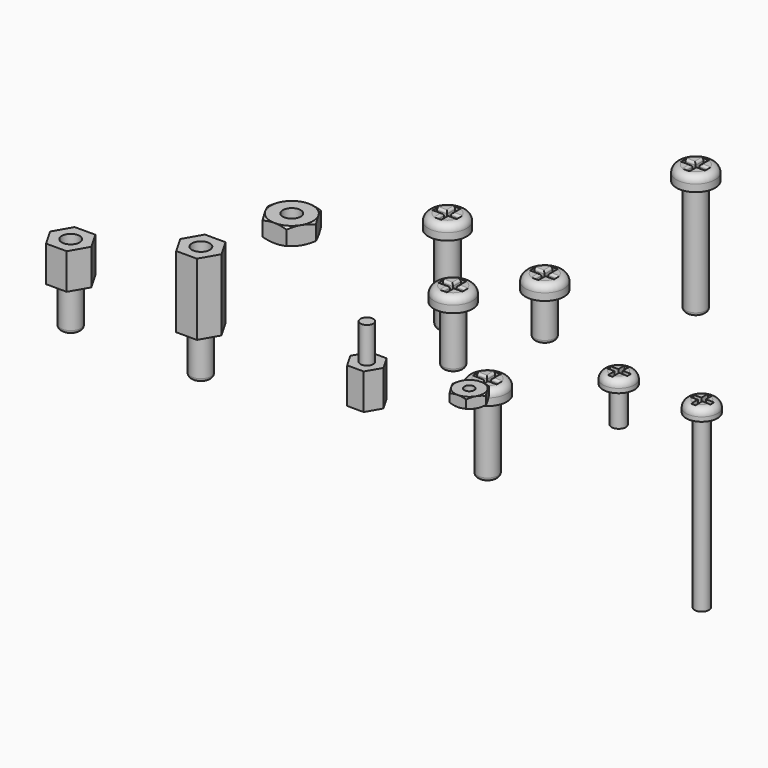
from build123d import *

# Parameters (mm, degrees)
F0_R        = 1.25
F1_DEPTH    = 2.5
F2_R        = 2.7
F3_DEPTH    = 2
F4_R        = 1
F6_DEPTH    = 1
F7_T1_DEPTH = 2.1580906364
F7_T3_DEPTH = 2.1580906364
F7_T5_DEPTH = 2.1580906364
F7_T7_DEPTH = 2.1580906364
F8_R        = 1.45
F13_DEPTH   = 12
F14_R       = 0.5
F15_R       = 1.45
F16_DEPTH   = 6
F17_R       = 0.5
F20_R       = 1.45
F21_DEPTH   = 10
F22_R       = 0.5
F23_R       = 1.45
F24_DEPTH   = 8
F25_R       = 0.5
F27_DEPTH   = 10
F28_R       = 1.25
F29_DEPTH   = 7.38
F30_R       = 1.45
F31_DEPTH   = 6
F32_R       = 0.5
F39_R       = 0.75
F40_DEPTH   = 5
F41_R       = 0.9
F41_R_2     = 0.75
F42_DEPTH   = 5
F43_R       = 0.7
F44_DEPTH   = 1.5
F45_R       = 2.2
F46_DEPTH   = 1.6
F48_DEPTH   = 1
F51_R       = 1
F52_DEPTH   = 5
F54_R       = 7.4954370555
F54_R_2     = 1.25
F55_DEPTH   = 5
F56_R       = 1
F57_DEPTH   = 24
F64_R       = 1.45
F65_DEPTH   = 16
F66_R       = 0.5


# Not quite as in the source:
# - a fillet or chamfer that OpenCascade refuses, or shapes differently, is made with other operations: its cross-section is extruded or revolved along the edge and cut away or added


with BuildPart() as f1:
    # F0 (on Top) → F1 (new body)
    with BuildSketch(Plane.XY):
        Polygon((-50.9010210277, 27.3592374967), (-49.1410704475, 30.2757263598), (-50.7868486027, 33.2581327032), (-54.1925773381, 33.3240501835), (-55.9525279183, 30.4075613204), (-54.3067497631, 27.425154977), align=None)
        with Locations((-52.5467991829, 30.3416438401)):
            Circle(F0_R, mode=Mode.SUBTRACT)
    extrude(amount=F1_DEPTH)

    # F37 (on 3pt) → F38 (revolve, cut)
    with BuildSketch(Plane(origin=(-0.6049917377, -1.0025575065, 0), x_dir=(-0.8561876086, 0.5166650549, 0), z_dir=(0.5166650549, 0.8561876086, 0))):
        Polygon((65.9979552705, 2.5), (63.6163854101, 2.5), (65.9979552705, 1.125), align=None)
        Polygon((65.9979552705, 0), (65.9979552705, 1.125), (63.6163854101, 0), align=None)
    revolve(axis=Axis((-52.5467991829, 30.3416438401, 2.5), (0, 0, 1)), mode=Mode.SUBTRACT)


with BuildPart() as f3:
    # F2 (on Top) → F3 (new body)
    with BuildSketch(Plane.XY):
        with Locations((-39.9160310626, 41.7706146836)):
            Circle(F2_R)
    extrude(amount=F3_DEPTH)

    # F4
    f4_edges = [f3.edges().sort_by_distance(p)[0] for p in [
        (-42.616031, 41.770615, 2),
    ]]
    fillet(f4_edges, radius=F4_R)

    # F5 (on face) → F6 (cut)
    with BuildSketch(Plane.XY.offset(2)):
        Polygon((-39.645745744, 43.4489906387), (-40.1863163812, 43.4489906387), (-40.1863163812, 42.0409000023), (-41.5944070177, 42.0409000023), (-41.5944070177, 41.500329365), (-40.1863163812, 41.500329365), (-40.1863163812, 40.0922387286), (-39.645745744, 40.0922387286), (-39.645745744, 41.500329365), (-38.2376551075, 41.500329365), (-38.2376551075, 42.0409000023), (-39.645745744, 42.0409000023), align=None)
    extrude(amount=-F6_DEPTH, mode=Mode.SUBTRACT)

    # F7: fillet of radius 0.3 on 8 edges, made by hand

    # F7_s2 → F7_t1 (cut)
    with BuildSketch(Plane.YZ.offset(-40.395745744)):
        with BuildLine():
            ThreePointArc((42.3409000023, 2), (42.1287679679, 1.9121320344), (42.0409000023, 1.7))
            Line((42.0409000023, 1.7), (42.0409000023, 2))
            Line((42.0409000023, 2), (42.3409000023, 2))
        make_face()
        with BuildLine():
            ThreePointArc((41.200329365, 2), (41.4124613994, 1.9121320344), (41.500329365, 1.7))
            Line((41.500329365, 1.7), (41.500329365, 2))
            Line((41.500329365, 2), (41.200329365, 2))
        make_face()
    extrude(amount=F7_T1_DEPTH, mode=Mode.SUBTRACT)

    # F7_s4 → F7_t3 (cut)
    with BuildSketch(Plane.XZ.offset(-43.4489906387)):
        with BuildLine():
            ThreePointArc((-39.345745744, 2), (-39.5578777783, 1.9121320344), (-39.645745744, 1.7))
            Line((-39.645745744, 1.7), (-39.645745744, 2))
            Line((-39.645745744, 2), (-39.345745744, 2))
        make_face()
        with BuildLine():
            ThreePointArc((-40.4863163812, 2), (-40.2741843469, 1.9121320344), (-40.1863163812, 1.7))
            Line((-40.1863163812, 1.7), (-40.1863163812, 2))
            Line((-40.1863163812, 2), (-40.4863163812, 2))
        make_face()
    extrude(amount=F7_T3_DEPTH, mode=Mode.SUBTRACT)

    # F7_s6 → F7_t5 (cut)
    with BuildSketch(Plane.YZ.offset(-41.5944070177)):
        with BuildLine():
            ThreePointArc((42.3409000023, 2), (42.1287679679, 1.9121320344), (42.0409000023, 1.7))
            Line((42.0409000023, 1.7), (42.0409000023, 2))
            Line((42.0409000023, 2), (42.3409000023, 2))
        make_face()
        with BuildLine():
            ThreePointArc((41.200329365, 2), (41.4124613994, 1.9121320344), (41.500329365, 1.7))
            Line((41.500329365, 1.7), (41.500329365, 2))
            Line((41.500329365, 2), (41.200329365, 2))
        make_face()
    extrude(amount=F7_T5_DEPTH, mode=Mode.SUBTRACT)

    # F7_s8 → F7_t7 (cut)
    with BuildSketch(Plane.XZ.offset(-42.250329365)):
        with BuildLine():
            ThreePointArc((-40.4863163812, 2), (-40.2741843469, 1.9121320344), (-40.1863163812, 1.7))
            Line((-40.1863163812, 1.7), (-40.1863163812, 2))
            Line((-40.1863163812, 2), (-40.4863163812, 2))
        make_face()
        with BuildLine():
            ThreePointArc((-39.345745744, 2), (-39.5578777783, 1.9121320344), (-39.645745744, 1.7))
            Line((-39.645745744, 1.7), (-39.645745744, 2))
            Line((-39.645745744, 2), (-39.345745744, 2))
        make_face()
    extrude(amount=F7_T7_DEPTH, mode=Mode.SUBTRACT)


with BuildPart() as f9_1:
    # F9: copy of F3
    add(f3.part.moved(Location((13.6, 0, -3))))


with BuildPart() as f10_1:
    # F10: copy of F9_1
    add(f9_1.part.moved(Location((-3.2, 30.4, 0))))

    # F64 (on face) → F65 (join)
    with BuildSketch(Plane(origin=(0, 0, -3), x_dir=(1, 0, 0), z_dir=(0, 0, -1))):
        with Locations((-29.5160310626, -72.1706146836)):
            Circle(F64_R)
    extrude(amount=F65_DEPTH)

    # F66
    f66_edges = [f10_1.edges().sort_by_distance(p)[0] for p in [
        (-30.966031, 72.170615, -19),
    ]]
    fillet(f66_edges, radius=F66_R)


with BuildPart() as f11_1:
    # F11: copy of F3
    add(f3.part.moved(Location((16.3, -46.7, 0))))


with BuildPart() as f12_1:
    # F12: copy of F3
    add(f3.part.moved(Location((11.2, -13, 0))))

    # F23 (on face) → F24 (join)
    with BuildSketch(Plane(origin=(0, 0, 0), x_dir=(1, 0, 0), z_dir=(0, 0, -1))):
        with Locations((-28.7160310626, -28.7706146836)):
            Circle(F23_R)
    extrude(amount=F24_DEPTH)

    # F25
    f25_edges = [f12_1.edges().sort_by_distance(p)[0] for p in [
        (-30.166031, 28.770615, -8),
    ]]
    fillet(f25_edges, radius=F25_R)


with BuildPart() as f3_1:
    add(f3.part)

    # F8 (on face) → F13 (join)
    with BuildSketch(Plane(origin=(0, 0, 0), x_dir=(1, 0, 0), z_dir=(0, 0, -1))):
        with Locations((-39.9160310626, -41.7706146836)):
            Circle(F8_R)
    extrude(amount=F13_DEPTH)

    # F14
    f14_edges = [f3_1.edges().sort_by_distance(p)[0] for p in [
        (-41.366031, 41.770615, -12),
    ]]
    fillet(f14_edges, radius=F14_R)


with BuildPart() as f9_1_1:
    add(f9_1.part)

    # F15 (on face) → F16 (join)
    with BuildSketch(Plane(origin=(0, 0, -3), x_dir=(1, 0, 0), z_dir=(0, 0, -1))):
        with Locations((-26.3160310626, -41.7706146836)):
            Circle(F15_R)
    extrude(amount=F16_DEPTH)

    # F17
    f17_edges = [f9_1_1.edges().sort_by_distance(p)[0] for p in [
        (-27.766031, 41.770615, -9),
    ]]
    fillet(f17_edges, radius=F17_R)


with BuildPart() as f11_1_1:
    # F18: moved
    add(f11_1.part.moved(Location((7.2, 0, 30.6))))


with BuildPart() as f11_1_2:
    # F19: moved
    add(f11_1_1.part.moved(Location((-1.9, 26.7, -35.8))))

    # F20 (on face) → F21 (join)
    with BuildSketch(Plane(origin=(0, 0, -5.2), x_dir=(1, 0, 0), z_dir=(0, 0, -1))):
        with Locations((-18.3160310626, -21.7706146836)):
            Circle(F20_R)
    extrude(amount=F21_DEPTH)

    # F22
    f22_edges = [f11_1_2.edges().sort_by_distance(p)[0] for p in [
        (-19.766031, 21.770615, -15.2),
    ]]
    fillet(f22_edges, radius=F22_R)


with BuildPart() as f27:
    # F26 (on Top) → F27 (new body)
    with BuildSketch(Plane.XY):
        Polygon((-44.9484995911, 4.2532703688), (-43.5051239182, 6.7532703688), (-44.9484995911, 9.2532703688), (-47.8352509371, 9.2532703688), (-49.2786266101, 6.7532703688), (-47.8352509371, 4.2532703688), align=None)
    extrude(amount=F27_DEPTH)

    # F28 (on face) → F29 (cut)
    with BuildSketch(Plane.XY.offset(10)):
        with Locations((-46.3918752641, 6.7532703688)):
            Circle(F28_R)
    extrude(amount=-F29_DEPTH, mode=Mode.SUBTRACT)

    # F30 (on face) → F31 (join)
    with BuildSketch(Plane(origin=(0, 0, 0), x_dir=(1, 0, 0), z_dir=(0, 0, -1))):
        with Locations((-46.3918752641, -6.7532703688)):
            Circle(F30_R)
    extrude(amount=F31_DEPTH)

    # F32
    f32_edges = [f27.edges().sort_by_distance(p)[0] for p in [
        (-47.841875, 6.75327, -6),
    ]]
    fillet(f32_edges, radius=F32_R)


with BuildPart() as f40:
    # F39 (on Top) → F40 (new body)
    with BuildSketch(Plane.XY):
        Polygon((-20.0601718143, 2.3061985367), (-18.9054712759, 4.3061985367), (-20.0601718143, 6.3061985367), (-22.3695728911, 6.3061985367), (-23.5242734295, 4.3061985367), (-22.3695728911, 2.3061985367), align=None)
        with Locations((-21.2148723527, 4.3061985367)):
            Circle(F39_R, mode=Mode.SUBTRACT)
    extrude(amount=F40_DEPTH)

    # F41 (on face) → F42 (join)
    with BuildSketch(Plane.XY.offset(5)):
        with Locations((-21.2148723527, 4.3061985367)):
            Circle(F41_R)
        with Locations((-21.2148723527, 4.3061985367)):
            Circle(F41_R_2, mode=Mode.SUBTRACT)
        with Locations((-21.2148723527, 4.3061985367)):
            Circle(F41_R_2)
    extrude(amount=F42_DEPTH)


with BuildPart() as f44:
    # F43 (on Top) → F44 (new body)
    with BuildSketch(Plane.XY):
        Polygon((-11.6123360878, 9.6400680006), (-10.4576355494, 11.6400680006), (-11.6123360878, 13.6400680006), (-13.9217371645, 13.6400680006), (-15.0764377029, 11.6400680006), (-13.9217371645, 9.6400680006), align=None)
        with Locations((-12.7670366262, 11.6400680006)):
            Circle(F43_R, mode=Mode.SUBTRACT)
    extrude(amount=F44_DEPTH)

    # F62 (on 3pt) → F63 (revolve, cut)
    with BuildSketch(Plane(origin=(-8.2320564517, 14.2583400251, 0), x_dir=(-0.8660254038, -0.5, 0), z_dir=(-0.5, 0.8660254038, 0))):
        Polygon((1.9375059433, 0.75), (3.236544049, 1.5), (1.9375059433, 1.5), align=None)
        Polygon((3.236544049, 0), (1.9375059433, 0.75), (1.9375059433, 0), align=None)
    revolve(axis=Axis((-12.7670366262, 11.6400680006, 1.5), (0, 0, 1)), mode=Mode.SUBTRACT)


with BuildPart() as f46:
    # F45 (on Top) → F46 (new body)
    with BuildSketch(Plane.XY):
        with Locations((-2.4725666735, 24.8899627477)):
            Circle(F45_R)
    extrude(amount=F46_DEPTH)

    # F47 (on face) → F48 (cut)
    with BuildSketch(Plane.XY.offset(1.6)):
        Polygon((-2.1590052638, 24.576401338), (-1.0345844785, 24.576401338), (-1.0345844785, 25.2035241574), (-2.1590052638, 25.2035241574), (-2.1590052638, 26.3279449428), (-2.7861280832, 26.3279449428), (-2.7861280832, 25.2035241574), (-3.9105488686, 25.2035241574), (-3.9105488686, 24.576401338), (-2.7861280832, 24.576401338), (-2.7861280832, 23.4519805526), (-2.1590052638, 23.4519805526), align=None)
    extrude(amount=-F48_DEPTH, mode=Mode.SUBTRACT)

    # F49: fillet of radius 1 on 1 edges, made by hand

    # F49_s1 → F49_t2 (revolve, cut)
    with BuildSketch(Plane.XZ.offset(-24.8899627477)):
        with BuildLine():
            ThreePointArc((-0.2725666735, 0.6), (-0.5654598923, 1.3071067812), (-1.2725666735, 1.6))
            Line((-1.2725666735, 1.6), (-0.2725666735, 1.6))
            Line((-0.2725666735, 1.6), (-0.2725666735, 0.6))
        make_face()
    revolve(axis=Axis((-2.4725666735, 24.8899627477, 1.6), (0, 0, 1)), mode=Mode.SUBTRACT)


with BuildPart() as f50_1:
    # F50: copy of F46
    add(f46.part.moved(Location((11.3, 0.4, 0))))

    # F56 (on face) → F57 (join)
    with BuildSketch(Plane(origin=(0, 0, 0), x_dir=(1, 0, 0), z_dir=(0, 0, -1))):
        with Locations((8.8274333265, -25.2899627477)):
            Circle(F56_R)
    extrude(amount=F57_DEPTH)


with BuildPart() as f46_1:
    add(f46.part)

    # F51 (on face) → F52 (join)
    with BuildSketch(Plane(origin=(0, 0, 0), x_dir=(1, 0, 0), z_dir=(0, 0, -1))):
        with Locations((-2.4725666735, -24.8899627477)):
            Circle(F51_R)
    extrude(amount=F52_DEPTH)


with BuildPart() as f53_1:
    # F53: copy of F27
    add(f27.part.moved(Location((-18.2, 0, 0))))

    # F54 (on face) → F55 (cut)
    with BuildSketch(Plane.XY.offset(10)):
        with Locations((-64.5918752641, 6.7532703688)):
            Circle(F54_R)
        Polygon((-66.0352509371, 4.2532703688), (-67.4786266101, 6.7532703688), (-66.0352509371, 9.2532703688), (-63.1484995911, 9.2532703688), (-61.7051239182, 6.7532703688), (-63.1484995911, 4.2532703688), align=None, mode=Mode.SUBTRACT)
        Polygon((-66.0352509371, 9.2532703688), (-67.4786266101, 6.7532703688), (-66.0352509371, 4.2532703688), (-63.1484995911, 4.2532703688), (-61.7051239182, 6.7532703688), (-63.1484995911, 9.2532703688), align=None)
        with Locations((-64.5918752641, 6.7532703688)):
            Circle(F54_R_2, mode=Mode.SUBTRACT)
    extrude(amount=-F55_DEPTH, mode=Mode.SUBTRACT)


solid = Compound([f1.part, f10_1.part, f12_1.part, f3_1.part, f9_1_1.part, f11_1_2.part, f27.part, f40.part, f44.part, f50_1.part, f46_1.part, f53_1.part])
